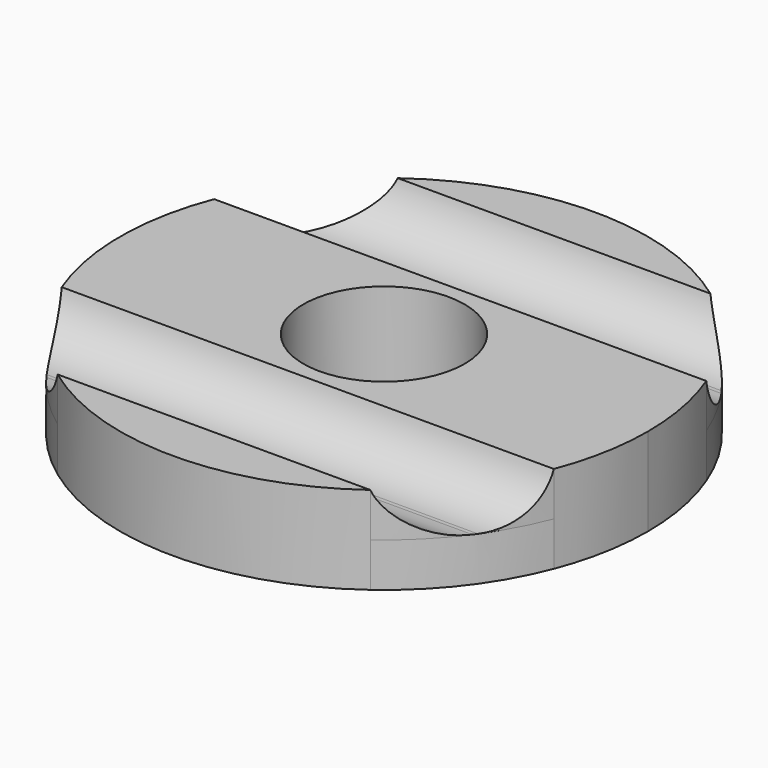
from build123d import *

# Parameters (mm, degrees)
F0_R         = 2.75
F1_DEPTH     = 3
F2_DEPTH     = 1.5
F3_T4_DEPTH  = 26.4678686971
F3_S5_R      = 9
F3_T6_DEPTH  = 15
F3_T10_DEPTH = 20.3478228694
F3_S11_R     = 9
F3_T12_DEPTH = 12
F3_T16_DEPTH = 26.4678686971
F3_S17_R     = 9
F3_T18_DEPTH = 15
F3_T22_DEPTH = 20.3478228694
F3_S23_R     = 9
F3_T24_DEPTH = 12


# Not quite as in the source:
# - a fillet or chamfer that OpenCascade refuses, or shapes differently, is made with other operations: its cross-section is extruded or revolved along the edge and cut away or added


with BuildPart() as f1:
    # F0 (on Top) → F1 (new body)
    with BuildSketch(Plane.XY):
        with BuildLine():
            Line((-5.3326822519, 7.25), (5.3326822519, 7.25))
            ThreePointArc((5.3326822519, 7.25), (0, 9), (-5.3326822519, 7.25))
        make_face()
        with BuildLine():
            Line((-8.3927051658, 3.25), (8.3927051658, 3.25))
            ThreePointArc((8.3927051658, 3.25), (7.1481861295, 5.4684033372), (5.3326822519, 7.25))
            Line((5.3326822519, 7.25), (-5.3326822519, 7.25))
            ThreePointArc((-5.3326822519, 7.25), (-7.1481861295, 5.4684033372), (-8.3927051658, 3.25))
        make_face()
        with BuildLine():
            ThreePointArc((5.3326822519, -7.25), (7.1481861295, -5.4684033372), (8.3927051658, -3.25))
            Line((8.3927051658, -3.25), (-8.3927051658, -3.25))
            ThreePointArc((-8.3927051658, -3.25), (-7.1481861295, -5.4684033372), (-5.3326822519, -7.25))
            Line((-5.3326822519, -7.25), (5.3326822519, -7.25))
        make_face()
        with BuildLine():
            ThreePointArc((-5.3326822519, -7.25), (0, -9), (5.3326822519, -7.25))
            Line((5.3326822519, -7.25), (-5.3326822519, -7.25))
        make_face()
        with BuildLine():
            ThreePointArc((8.3927051658, -3.25), (8.8468736425, -1.6531263575), (9, 0))
            ThreePointArc((9, 0), (8.8468736425, 1.6531263575), (8.3927051658, 3.25))
            Line((8.3927051658, 3.25), (-8.3927051658, 3.25))
            ThreePointArc((-8.3927051658, 3.25), (-9, 0), (-8.3927051658, -3.25))
            Line((-8.3927051658, -3.25), (8.3927051658, -3.25))
        make_face()
        Circle(F0_R, mode=Mode.SUBTRACT)
    extrude(amount=-F1_DEPTH)

    # F0 (on Top) → F2 (cut)
    with BuildSketch(Plane.XY):
        with BuildLine():
            Line((-8.3927051658, 3.25), (8.3927051658, 3.25))
            ThreePointArc((8.3927051658, 3.25), (7.1481861295, 5.4684033372), (5.3326822519, 7.25))
            Line((5.3326822519, 7.25), (-5.3326822519, 7.25))
            ThreePointArc((-5.3326822519, 7.25), (-7.1481861295, 5.4684033372), (-8.3927051658, 3.25))
        make_face()
        with BuildLine():
            ThreePointArc((5.3326822519, -7.25), (7.1481861295, -5.4684033372), (8.3927051658, -3.25))
            Line((8.3927051658, -3.25), (-8.3927051658, -3.25))
            ThreePointArc((-8.3927051658, -3.25), (-7.1481861295, -5.4684033372), (-5.3326822519, -7.25))
            Line((-5.3326822519, -7.25), (5.3326822519, -7.25))
        make_face()
    extrude(amount=-F2_DEPTH, mode=Mode.SUBTRACT)

    # F3: fillet of radius 2 on 4 edges, made by hand


with BuildPart() as f3_tool2:
    # F3_s3 → F3_t4 (new body)
    with BuildSketch(Plane.YZ.offset(-13.2339343486)):
        with BuildLine():
            ThreePointArc((3.25, 0), (3.9617468017, -1.0811388301), (5.1864916731, -1.5))
            Line((5.1864916731, -1.5), (3.25, -1.5))
            Line((3.25, -1.5), (3.25, 0))
        make_face()
    extrude(amount=F3_T4_DEPTH)

    # F3_s5 → F3_t6 (intersect, symmetric)
    with BuildSketch(Plane.XY.offset(-0.8)):
        Circle(F3_S5_R)
    extrude(amount=F3_T6_DEPTH, both=True, mode=Mode.INTERSECT)


with BuildPart() as f1_1:
    add(f1.part)

    # F3_t1: union F3_tool2
    add(f3_tool2.part)


with BuildPart() as f3_tool8:
    # F3_s9 → F3_t10 (new body)
    with BuildSketch(Plane.YZ.offset(10.1739114347)):
        with BuildLine():
            ThreePointArc((5.3135083269, -1.5), (6.5382531983, -1.0811388301), (7.25, 0))
            Line((7.25, 0), (7.25, -1.5))
            Line((7.25, -1.5), (5.3135083269, -1.5))
        make_face()
    extrude(amount=-F3_T10_DEPTH)

    # F3_s11 → F3_t12 (intersect, symmetric)
    with BuildSketch(Plane.XY.offset(-0.8)):
        Circle(F3_S11_R)
    extrude(amount=F3_T12_DEPTH, both=True, mode=Mode.INTERSECT)


with BuildPart() as f1_2:
    add(f1_1.part)

    # F3_t7: union F3_tool8
    add(f3_tool8.part)


with BuildPart() as f3_tool14:
    # F3_s15 → F3_t16 (new body)
    with BuildSketch(Plane.YZ.offset(13.2339343486)):
        with BuildLine():
            ThreePointArc((-3.25, 0), (-3.9617468017, -1.0811388301), (-5.1864916731, -1.5))
            Line((-5.1864916731, -1.5), (-3.25, -1.5))
            Line((-3.25, -1.5), (-3.25, 0))
        make_face()
    extrude(amount=-F3_T16_DEPTH)

    # F3_s17 → F3_t18 (intersect, symmetric)
    with BuildSketch(Plane.XY.offset(-0.8)):
        Circle(F3_S17_R)
    extrude(amount=F3_T18_DEPTH, both=True, mode=Mode.INTERSECT)


with BuildPart() as f1_3:
    add(f1_2.part)

    # F3_t13: union F3_tool14
    add(f3_tool14.part)


with BuildPart() as f3_tool20:
    # F3_s21 → F3_t22 (new body)
    with BuildSketch(Plane.YZ.offset(-10.1739114347)):
        with BuildLine():
            ThreePointArc((-5.3135083269, -1.5), (-6.5382531983, -1.0811388301), (-7.25, 0))
            Line((-7.25, 0), (-7.25, -1.5))
            Line((-7.25, -1.5), (-5.3135083269, -1.5))
        make_face()
    extrude(amount=F3_T22_DEPTH)

    # F3_s23 → F3_t24 (intersect, symmetric)
    with BuildSketch(Plane.XY.offset(-0.8)):
        Circle(F3_S23_R)
    extrude(amount=F3_T24_DEPTH, both=True, mode=Mode.INTERSECT)


with BuildPart() as f1_4:
    add(f1_3.part)

    # F3_t19: union F3_tool20
    add(f3_tool20.part)


solid = f1_4.part
